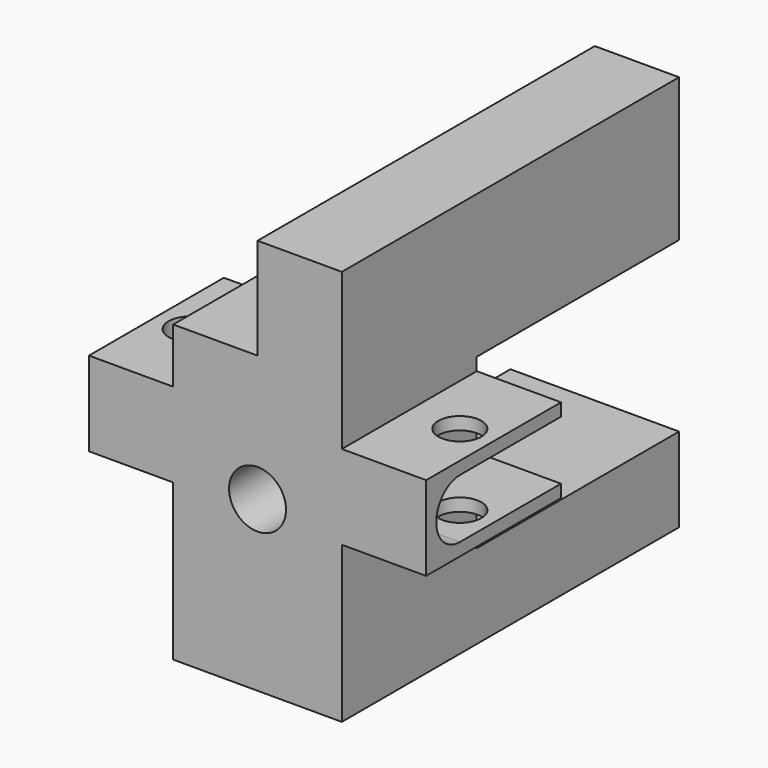
from build123d import *

# Parameters (mm, degrees)
F1_DEPTH = 25
F3_D     = 6.7564
F4_W     = 69.7505115181
F4_H     = 20
F5_DEPTH = 40.001
F7_DEPTH = 10
F9_D     = 5.1054


# Not quite as in the source:
# - a feature names something its author has since deleted; it is built from what else it names


with BuildPart() as f1:
    # F0 (on Front) → F1 (new body, symmetric)
    with BuildSketch(Plane.XZ):
        Polygon((10, 27), (0, 27), (0, 15), (-10, 15), (-10, 8.5), (-20, 8.5), (-20, -1.5), (-10, -1.5), (-10, -20), (10, -20), (10, -1.5), (20, -1.5), (20, 8.5), (10, 8.5), align=None)
    extrude(amount=F1_DEPTH, both=True)

    # F3 (through all)
    with Locations(Plane.XZ.offset(25)):
        with Locations((0, 0)):
            Hole(F3_D / 2)

    # F4 (on face) → F5 (cut, through all)
    with BuildSketch(Plane.YZ.offset(20)):
        with Locations((29.875255759, 0)):
            Rectangle(F4_W, F4_H)
    extrude(amount=-F5_DEPTH, mode=Mode.SUBTRACT)

    # F6 (on face) → F7 (cut)
    with BuildSketch(Plane.YZ.offset(20)):
        with BuildLine():
            ThreePointArc((-20, 7), (-23.5, 3.5), (-20, 0))
            Line((-20, 0), (-5, 0))
            Line((-5, 0), (-5, 7))
            Line((-5, 7), (-20, 7))
        make_face()
    extrude(amount=-F7_DEPTH, mode=Mode.SUBTRACT)

    # F9 (through all)
    with Locations(Plane.XY.offset(8.5)):
        with Locations((16, -15), (-16, -15)):
            Hole(F9_D / 2)


solid = f1.part
